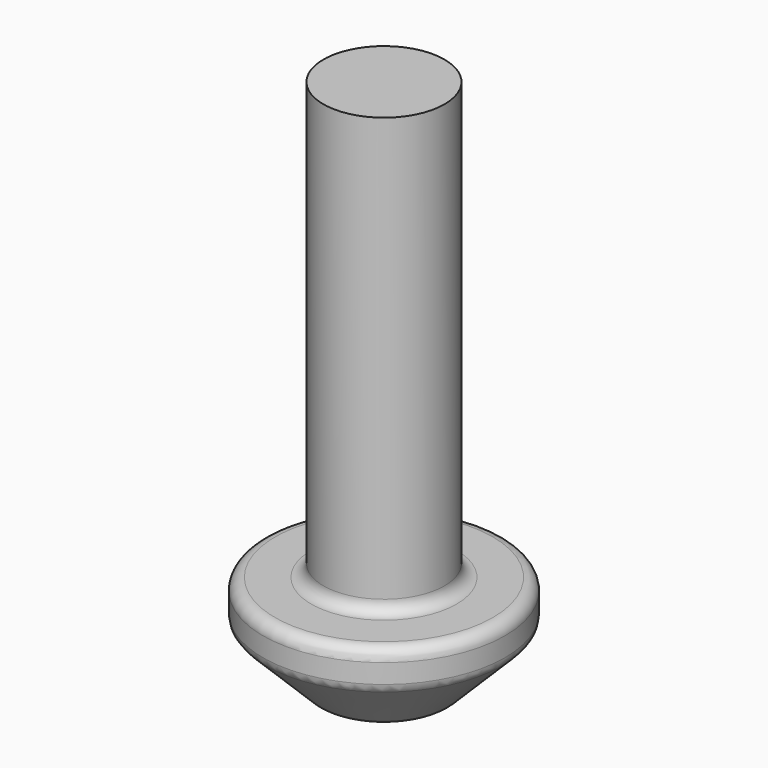
from build123d import *

# Parameters (mm, degrees)
F1_R     = 2.5
F1_R_2   = 1.25
F2_DEPTH = 2
F3_START = 1.5
F3_DEPTH = 0.5
F4_START = 2
F4_DEPTH = 9
F5_SIZE2 = 1.25
F5_SIZE  = 1.25
F6_R     = 0.25


# Not quite as in the source:
# - a feature names something its author has since deleted; it is built from what else it names


with BuildPart() as f2:
    # F1 (on Top) → F2 (new body)
    with BuildSketch(Plane.XY):
        Circle(F1_R)
        Circle(F1_R_2, mode=Mode.SUBTRACT)
        Circle(F1_R_2)
        Polygon((-0.4330127019, -0.75), (-0.8660254038, 0), (-0.4330127019, 0.75), (0.4330127019, 0.75), (0.8660254038, 0), (0.4330127019, -0.75), align=None, mode=Mode.SUBTRACT)
    extrude(amount=F2_DEPTH)

    # F1 (on Top) → F3 (join)
    with BuildSketch(Plane.XY.offset(F3_START)):
        Polygon((-0.4330127019, 0.75), (-0.8660254038, 0), (-0.4330127019, -0.75), (0.4330127019, -0.75), (0.8660254038, 0), (0.4330127019, 0.75), align=None)
    extrude(amount=F3_DEPTH)

    # F1 (on Top) → F4 (join)
    with BuildSketch(Plane.XY.offset(F4_START)):
        Circle(F1_R_2)
        Polygon((-0.4330127019, -0.75), (-0.8660254038, 0), (-0.4330127019, 0.75), (0.4330127019, 0.75), (0.8660254038, 0), (0.4330127019, -0.75), align=None, mode=Mode.SUBTRACT)
        Polygon((-0.4330127019, 0.75), (-0.8660254038, 0), (-0.4330127019, -0.75), (0.4330127019, -0.75), (0.8660254038, 0), (0.4330127019, 0.75), align=None)
    extrude(amount=F4_DEPTH)

    # F5
    f5_edges = [f2.edges().sort_by_distance(p)[0] for p in [
        (-2.5, 0, 0),
    ]]
    chamfer(f5_edges, length=F5_SIZE, length2=F5_SIZE2)

    # F6
    f6_edges = [f2.edges().sort_by_distance(p)[0] for p in [
        (-2.5, 0, 2),
        (-1.25, 0, 2),
        (-1.25, 0, 0),
        (-2.5, 0, 1.25),
    ]]
    fillet(f6_edges, radius=F6_R)


solid = f2.part
